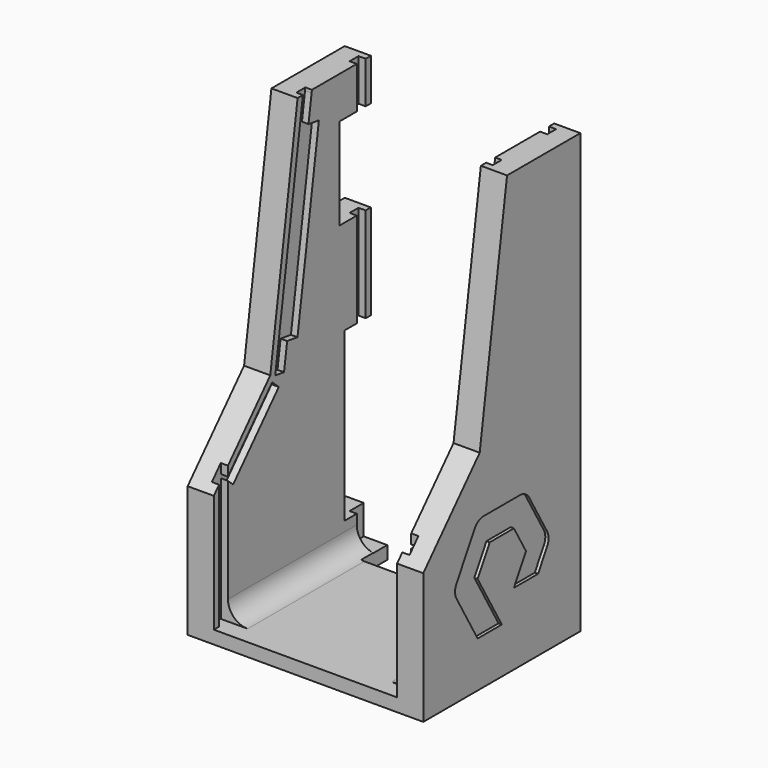
from build123d import *

# Parameters (mm, degrees)
F1_DEPTH     = 18
F2_W         = 30
F2_H         = 80
F3_DEPTH     = 14
F4_W         = 5
F4_H         = 25.6
F4_W_2       = 6
F4_H_2       = 14
F5_DEPTH     = 25
F6_W         = 5
F6_H         = 5
F7_DEPTH     = 11.5
F8_W         = 10
F8_H         = 10
F9_DEPTH     = 15.1
F10_W        = 1.7
F10_H        = 17.78
F10_H_2      = 10
F11_DEPTH    = 15.1
F13_DEPTH    = 15.1
F15_DEPTH    = 15
F17_DEPTH    = 0.5
F19_DEPTH    = 0.5
F20_T4_DEPTH = 32.1
F20_T9_DEPTH = 32.1
F21_T4_DEPTH = 32.1
F21_T9_DEPTH = 24.6


# Not quite as in the source:
# - a fillet or chamfer that OpenCascade refuses, or shapes differently, is made with other operations: its cross-section is extruded or revolved along the edge and cut away or added


with BuildPart() as f1:
    # F0 (on Right) → F1 (new body, symmetric)
    with BuildSketch(Plane.YZ):
        Polygon((-30, 0), (0, 0), (0, 67), (-14, 67), (-19.2224497622, 31.8255828978), (-30, 20), align=None)
    extrude(amount=F1_DEPTH, both=True)

    # F2 (on Right) → F3 (cut, symmetric)
    with BuildSketch(Plane.YZ):
        with Locations((-15, 42)):
            Rectangle(F2_W, F2_H)
    extrude(amount=F3_DEPTH, both=True, mode=Mode.SUBTRACT)

    # F4 (on Right) → F5 (cut)
    with BuildSketch(Plane.YZ):
        with Locations((-2.5, 19.3)):
            Rectangle(F4_W, F4_H)
        with Locations((-3, 53.6)):
            Rectangle(F4_W_2, F4_H_2)
    extrude(amount=-F5_DEPTH, mode=Mode.SUBTRACT)

    # F6 (on Right) → F7 (cut, symmetric)
    with BuildSketch(Plane.YZ):
        with Locations((-2.5, 2.5)):
            Rectangle(F6_W, F6_H)
    extrude(amount=F7_DEPTH, both=True, mode=Mode.SUBTRACT)

    # F8 (on Right) → F9 (cut, symmetric)
    with BuildSketch(Plane.YZ):
        Polygon((-2.7, 67), (-2.7, 2), (-1, 2), (-1, 12), (-1, 67), align=None)
        with Locations((4, 7)):
            Rectangle(F8_W, F8_H)
    extrude(amount=F9_DEPTH, both=True, mode=Mode.SUBTRACT)

    # F10 (on Right) → F11 (cut, symmetric)
    with BuildSketch(Plane.YZ):
        with Locations((-28.15, 10.89)):
            Rectangle(F10_W, F10_H)
        with Locations((-28.15, 24.78)):
            Rectangle(F10_W, F10_H_2)
    extrude(amount=F11_DEPTH, both=True, mode=Mode.SUBTRACT)

    # F12 (on Right) → F13 (cut, symmetric)
    with BuildSketch(Plane.YZ):
        Polygon((-17.5946665501, 29.6033232788), (-18.851134733, 30.7484379915), (-27.5769088442, 21.1741504379), (-26.3204406613, 20.0290357252), align=None)
    extrude(amount=F13_DEPTH, both=True, mode=Mode.SUBTRACT)

    # F14 (on Right) → F15 (cut, symmetric)
    with BuildSketch(Plane.YZ):
        Polygon((-11.9167287085, 62.6468424419), (-11.3292765417, 66.6034697875), (-13.0108431636, 66.8531369583), (-18.2705961384, 31.4274740197), (-16.5890295165, 31.1778068488), (-16.0015773498, 35.1344341944), align=None)
        Polygon((-13.0108431636, 66.8531369583), (-11.3292765417, 66.6034697875), (-9.8606461249, 76.4950381514), (-11.5422127468, 76.7447053223), align=None)
        Polygon((-9.9384150357, 62.3531163585), (-11.9167287085, 62.6468424419), (-16.0015773498, 35.1344341944), (-14.023263677, 34.840708111), align=None)
    extrude(amount=F15_DEPTH, both=True, mode=Mode.SUBTRACT)

    # F16 (on face) → F17 (cut)
    with BuildSketch(Plane.YZ.offset(18)):
        with BuildLine():
            Line((-19.6188021535, 7), (-15, 7))
            Line((-15, 7), (-17.3094010768, 11))
            Line((-17.3094010768, 11), (-19.6188021535, 15))
            Line((-19.6188021535, 15), (-17.3094010768, 19))
            Line((-17.3094010768, 19), (-12.6905989232, 19))
            Line((-12.6905989232, 19), (-10.3811978465, 15))
            Line((-10.3811978465, 15), (-12.6905989232, 11))
            Line((-12.6905989232, 11), (-8.0717967697, 11))
            Line((-8.0717967697, 11), (-6.3397459622, 14))
            ThreePointArc((-6.3397459622, 14), (-6.0717967697, 15), (-6.3397459622, 16))
            Line((-6.3397459622, 16), (-9.8038475773, 22))
            ThreePointArc((-9.8038475773, 22), (-10.5358983849, 22.7320508076), (-11.5358983849, 23))
            Line((-11.5358983849, 23), (-18.4641016151, 23))
            ThreePointArc((-18.4641016151, 23), (-19.4641016151, 22.7320508076), (-20.1961524227, 22))
            Line((-20.1961524227, 22), (-23.6602540378, 16))
            ThreePointArc((-23.6602540378, 16), (-23.9282032303, 15), (-23.6602540378, 14))
            Line((-23.6602540378, 14), (-19.6188021535, 7))
        make_face()
    extrude(amount=-F17_DEPTH, mode=Mode.SUBTRACT)

    # F18 (on face) → F19 (cut)
    with BuildSketch(Plane(origin=(-18, 0, 0), x_dir=(0, -1, 0), z_dir=(-1, 0, 0))):
        with BuildLine():
            Line((18.4641016151, 23), (11.5358983849, 23))
            ThreePointArc((11.5358983849, 23), (10.5358983849, 22.7320508076), (9.8038475773, 22))
            Line((9.8038475773, 22), (6.3397459622, 16))
            ThreePointArc((6.3397459622, 16), (6.0717967697, 15), (6.3397459622, 14))
            Line((6.3397459622, 14), (10.3811978465, 7))
            Line((10.3811978465, 7), (15, 7))
            Line((15, 7), (12.6905989232, 11))
            Line((12.6905989232, 11), (10.3811978465, 15))
            Line((10.3811978465, 15), (12.6905989232, 19))
            Line((12.6905989232, 19), (17.3094010768, 19))
            Line((17.3094010768, 19), (19.6188021535, 15))
            Line((19.6188021535, 15), (17.3094010768, 11))
            Line((17.3094010768, 11), (21.9282032303, 11))
            Line((21.9282032303, 11), (23.6602540378, 14))
            ThreePointArc((23.6602540378, 14), (23.9282032303, 15), (23.6602540378, 16))
            Line((23.6602540378, 16), (20.1961524227, 22))
            ThreePointArc((20.1961524227, 22), (19.4641016151, 22.7320508076), (18.4641016151, 23))
        make_face()
    extrude(amount=-F19_DEPTH, mode=Mode.SUBTRACT)

    # F20: fillet of radius 3 on 1 edges, made by hand


with BuildPart() as f20_tool2:
    # F20_s3 → F20_t4 (new body)
    with BuildSketch(Plane.XZ.offset(27.3)):
        with BuildLine():
            ThreePointArc((-14, 5), (-13.1213203436, 2.8786796564), (-11, 2))
            Line((-11, 2), (-14, 2))
            Line((-14, 2), (-14, 5))
        make_face()
    extrude(amount=-F20_T4_DEPTH)

    split(bisect_by=Plane.XZ.offset(5), keep=Keep.TOP)


with BuildPart() as f1_1:
    add(f1.part)

    # F20_t1: union F20_tool2
    add(f20_tool2.part)


with BuildPart() as f20_tool7:
    # F20_s8 → F20_t9 (new body)
    with BuildSketch(Plane.XZ.offset(34.8)):
        with BuildLine():
            ThreePointArc((-14, 5), (-13.1213203436, 2.8786796564), (-11, 2))
            Line((-11, 2), (-14, 2))
            Line((-14, 2), (-14, 5))
        make_face()
    extrude(amount=-F20_T9_DEPTH)

    split(bisect_by=Plane.YZ.offset(-11.5), keep=Keep.BOTTOM)

    split(bisect_by=Plane.XZ.offset(5), keep=Keep.BOTTOM)


with BuildPart() as f1_2:
    add(f1_1.part)

    # F20_t6: union F20_tool7
    add(f20_tool7.part)

    # F21: fillet of radius 3 on 1 edges, made by hand


with BuildPart() as f21_tool2:
    # F21_s3 → F21_t4 (new body)
    with BuildSketch(Plane.XZ.offset(27.3)):
        with BuildLine():
            ThreePointArc((11, 2), (13.1213203436, 2.8786796564), (14, 5))
            Line((14, 5), (14, 2))
            Line((14, 2), (11, 2))
        make_face()
    extrude(amount=-F21_T4_DEPTH)

    split(bisect_by=Plane.XZ.offset(5), keep=Keep.TOP)


with BuildPart() as f1_3:
    add(f1_2.part)

    # F21_t1: union F21_tool2
    add(f21_tool2.part)


with BuildPart() as f21_tool7:
    # F21_s8 → F21_t9 (new body)
    with BuildSketch(Plane.XZ.offset(27.3)):
        with BuildLine():
            ThreePointArc((11, 2), (13.1213203436, 2.8786796564), (14, 5))
            Line((14, 5), (14, 2))
            Line((14, 2), (11, 2))
        make_face()
    extrude(amount=-F21_T9_DEPTH)

    split(bisect_by=Plane.YZ.offset(11.5), keep=Keep.TOP)


with BuildPart() as f1_4:
    add(f1_3.part)

    # F21_t6: union F21_tool7
    add(f21_tool7.part)


solid = f1_4.part
